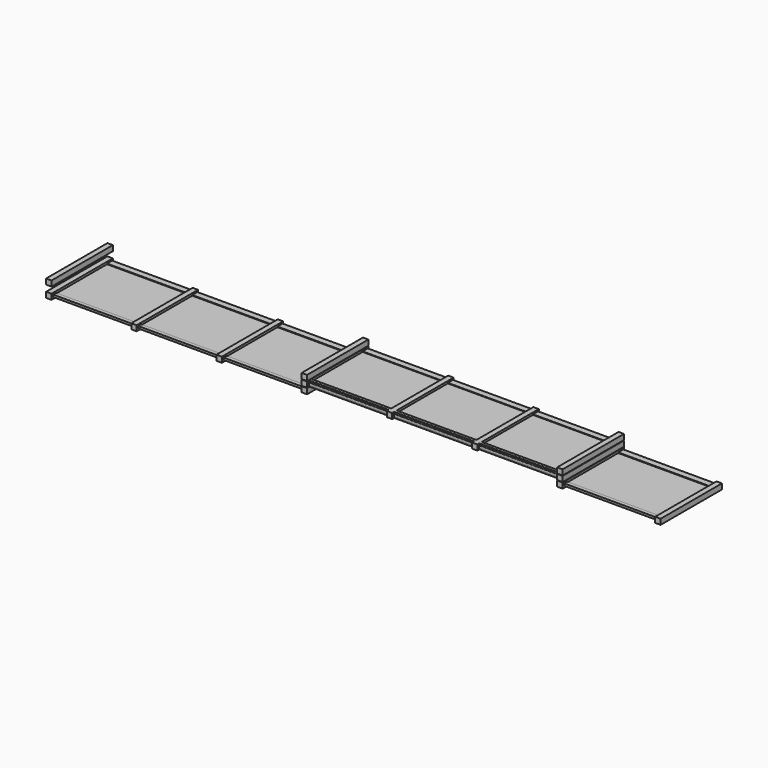
from build123d import *

# Parameters (mm, degrees)
F0_W        = 1873
F0_H        = 25
F0_W_2      = 63.5
F0_W_3      = 127
F0_H_2      = 51
F1_DEPTH    = 1800
F2_W        = 150
F2_H        = 50
F2_W_2      = 88
F3_DEPTH    = 6000
F4_DEPTH    = 50
F0_H_3      = 127
F5_DEPTH    = 1800
F0_H_4      = 22
F0_H_5      = 52.5
F0_W_4      = 2173
F6_W        = 150
F6_H        = 51
F6_W_2      = 88
F7_DEPTH    = 2370
F8_W        = 150
F8_H        = 51
F8_W_2      = 88
F9_DEPTH    = 6090
F7_FACE_W   = 2173
F7_FACE_H   = 50
F7_FACE_H_2 = 20
F9_FACE_W   = 1873
F9_FACE_H   = 50
F9_FACE_H_2 = 20
F10_DEPTH   = 50
F12_DEPTH   = 6000


# Not quite as in the source:
# - a feature names something its author has since deleted; it is built from what else it names


with BuildPart() as f1:
    # F0 (on Front) → F1 (new body)
    with BuildSketch(Plane.XZ):
        with Locations((-2076.5718817711, 0)):
            Rectangle(F0_W, F0_H)
        with Locations((-3044.8218817711, 0)):
            Rectangle(F0_W_2, F0_H)
        with Locations((-1076.5718817711, 0)):
            Rectangle(F0_W_3, F0_H)
        with Locations((-76.5718817711, 0)):
            Rectangle(F0_W, F0_H)
        with Locations((923.4281182289, 0)):
            Rectangle(F0_W_3, F0_H)
        with Locations((1923.4281182289, 0)):
            Rectangle(F0_W, F0_H)
        with Locations((2891.6781182289, 0)):
            Rectangle(F0_W_2, F0_H)
        Polygon((-3013.0718817711, -63.5), (-3013.0718817711, -12.5), (-3076.5718817711, -12.5), (-3076.5718817711, 12.5), (-3013.0718817711, 12.5), (-3013.0718817711, 63.5), (-3140.0718817711, 63.5), (-3140.0718817711, -63.5), align=None)
        with Locations((-1076.5718817711, -38)):
            Rectangle(F0_W_3, F0_H_2)
        with Locations((-1076.5718817711, 38)):
            Rectangle(F0_W_3, F0_H_2)
        with Locations((923.4281182289, -38)):
            Rectangle(F0_W_3, F0_H_2)
        with Locations((923.4281182289, 38)):
            Rectangle(F0_W_3, F0_H_2)
        Polygon((2923.4281182289, 12.5), (2923.4281182289, -12.5), (2859.9281182289, -12.5), (2859.9281182289, -63.5), (2986.9281182289, -63.5), (2986.9281182289, 63.5), (2859.9281182289, 63.5), (2859.9281182289, 12.5), align=None)
    extrude(amount=F1_DEPTH)

    # F2 (on face) → F3 (join)
    with BuildSketch(Plane(origin=(-3140.0718817711, 0, 0), x_dir=(0, -1, 0), z_dir=(-1, 0, 0))):
        with Locations((95, 0)):
            Rectangle(F2_W, F2_H)
        with Locations((1706, 0)):
            Rectangle(F2_W_2, F2_H)
    extrude(amount=-F3_DEPTH)

    # F4 (cut): faces of the model
    f4_faces = [f1.faces().sort_by_distance(p)[0] for p in [
        (1923.4281182289, -1775, 12.5),
        (-76.5718817711, -1775, 12.5),
        (-2076.5718817711, -1775, 12.5),
        (-2076.5718817711, -10, 12.5),
        (-76.5718817711, -10, 12.5),
        (1923.4281182289, -10, 12.5),
    ]]
    extrude(f4_faces, amount=-F4_DEPTH, mode=Mode.SUBTRACT)

    # F11 (on face) → F12 (join)
    with BuildSketch(Plane.YZ.offset(2986.9281182289)):
        with BuildLine():
            Line((-1668, -58.5), (-1668, -25.5))
            Line((-1668, -25.5), (-1744, -25.5))
            Line((-1744, -25.5), (-1744, -58.5))
            ThreePointArc((-1744, -58.5), (-1742.5355339059, -62.0355339059), (-1739, -63.5))
            Line((-1739, -63.5), (-1673, -63.5))
            ThreePointArc((-1673, -63.5), (-1669.4644660941, -62.0355339059), (-1668, -58.5))
        make_face()
        with BuildLine():
            Line((-1744, 25.5), (-1668, 25.5))
            Line((-1668, 25.5), (-1668, 58.5))
            ThreePointArc((-1668, 58.5), (-1669.4644660941, 62.0355339059), (-1673, 63.5))
            Line((-1673, 63.5), (-1739, 63.5))
            ThreePointArc((-1739, 63.5), (-1742.5355339059, 62.0355339059), (-1744, 58.5))
            Line((-1744, 58.5), (-1744, 25.5))
        make_face()
    extrude(amount=-F12_DEPTH)


with BuildPart() as f5:
    # F0 (on Front) → F5 (new body)
    with BuildSketch(Plane.XZ):
        with Locations((-3076.5718817711, 137)):
            Rectangle(F0_W_3, F0_H_3)
    extrude(amount=F5_DEPTH)


with BuildPart() as f5b:
    # F0 (on Front) → F5, piece 2 (new body)
    with BuildSketch(Plane.XZ):
        Polygon((-3140.0718817711, -200.5), (-3013.0718817711, -200.5), (-3013.0718817711, -73.5), (-3140.0718817711, -73.5), (-3140.0718817711, -126), (-3140.0718817711, -148), align=None)
        with Locations((-4076.5718817711, -137)):
            Rectangle(F0_W, F0_H_4)
        with Locations((-5076.5718817711, -174.25)):
            Rectangle(F0_W_3, F0_H_5)
        with Locations((-5076.5718817711, -137)):
            Rectangle(F0_W_3, F0_H_4)
        with Locations((-5076.5718817711, -99.75)):
            Rectangle(F0_W_3, F0_H_5)
        with Locations((-6076.5718817711, -137)):
            Rectangle(F0_W, F0_H_4)
        with Locations((-7076.5718817711, -174.25)):
            Rectangle(F0_W_3, F0_H_5)
        with Locations((-7076.5718817711, -137)):
            Rectangle(F0_W_3, F0_H_4)
        with Locations((-7076.5718817711, -99.75)):
            Rectangle(F0_W_3, F0_H_5)
        with Locations((-8076.5718817711, -137)):
            Rectangle(F0_W, F0_H_4)
        Polygon((-9013.0718817711, -200.5), (-9013.0718817711, -148), (-9013.0718817711, -126), (-9013.0718817711, -73.5), (-9140.0718817711, -73.5), (-9140.0718817711, -200.5), align=None)
    extrude(amount=F5_DEPTH)

    # F8 (on face) → F9 (join)
    with BuildSketch(Plane(origin=(-9140.0718817711, 0, 0), x_dir=(0, -1, 0), z_dir=(-1, 0, 0))):
        with Locations((95, -137)):
            Rectangle(F8_W, F8_H)
        with Locations((1706, -137)):
            Rectangle(F8_W_2, F8_H)
    extrude(amount=-F9_DEPTH)


with BuildPart() as f5c:
    # F0 (on Front) → F5, piece 3 (new body)
    with BuildSketch(Plane.XZ):
        with Locations((-9076.5718817711, 137)):
            Rectangle(F0_W_3, F0_H_3)
    extrude(amount=F5_DEPTH)


with BuildPart() as f5d:
    # F0 (on Front) → F5, piece 4 (new body)
    with BuildSketch(Plane.XZ):
        Polygon((2859.9281182289, -200.5), (2986.9281182289, -200.5), (2986.9281182289, -148), (2986.9281182289, -126), (2986.9281182289, -73.5), (2859.9281182289, -73.5), align=None)
        with Locations((4073.4281182289, -137)):
            Rectangle(F0_W_4, F0_H_4)
        Polygon((5159.9281182289, -126), (5159.9281182289, -148), (5159.9281182289, -200.5), (5286.9281182289, -200.5), (5286.9281182289, -73.5), (5159.9281182289, -73.5), align=None)
    extrude(amount=F5_DEPTH)

    # F6 (on face) → F7 (join)
    with BuildSketch(Plane.YZ.offset(5286.9281182289)):
        with Locations((-95, -137)):
            Rectangle(F6_W, F6_H)
        with Locations((-1706, -137)):
            Rectangle(F6_W_2, F6_H)
    extrude(amount=-F7_DEPTH)


with BuildPart() as f5e:
    # F0 (on Front) → F5, piece 5 (new body)
    with BuildSketch(Plane.XZ):
        with Locations((2923.4281182289, 137)):
            Rectangle(F0_W_3, F0_H_3)
    extrude(amount=F5_DEPTH)


with BuildPart() as f10_tool:
    # F7_face (on face) + F9_face (on face) → F10 (new body)
    with BuildSketch(Plane(origin=(4073.4281182289, -1775, -148), x_dir=(1, 0, 0), z_dir=(0, 0, -1))):
        Rectangle(F7_FACE_W, F7_FACE_H)
        with Locations((0, -1765)):
            Rectangle(F7_FACE_W, F7_FACE_H_2)
    with BuildSketch(Plane(origin=(-4076.5718817711, -1775, -148), x_dir=(1, 0, 0), z_dir=(0, 0, -1))):
        Rectangle(F9_FACE_W, F9_FACE_H)
        with Locations((-2000, 0)):
            Rectangle(F9_FACE_W, F9_FACE_H)
        with Locations((-4000, 0)):
            Rectangle(F9_FACE_W, F9_FACE_H)
        with Locations((-4000, -1765)):
            Rectangle(F9_FACE_W, F9_FACE_H_2)
        with Locations((-2000, -1765)):
            Rectangle(F9_FACE_W, F9_FACE_H_2)
        with Locations((0, -1765)):
            Rectangle(F9_FACE_W, F9_FACE_H_2)
    extrude(amount=-F10_DEPTH)


with BuildPart() as f5b_1:
    add(f5b.part)

    # F10: cut by f10_tool
    add(f10_tool.part, mode=Mode.SUBTRACT)


with BuildPart() as f5d_1:
    add(f5d.part)

    # F10: cut by f10_tool
    add(f10_tool.part, mode=Mode.SUBTRACT)


solid = Compound([f1.part, f5.part, f5c.part, f5e.part, f5b_1.part, f5d_1.part])
